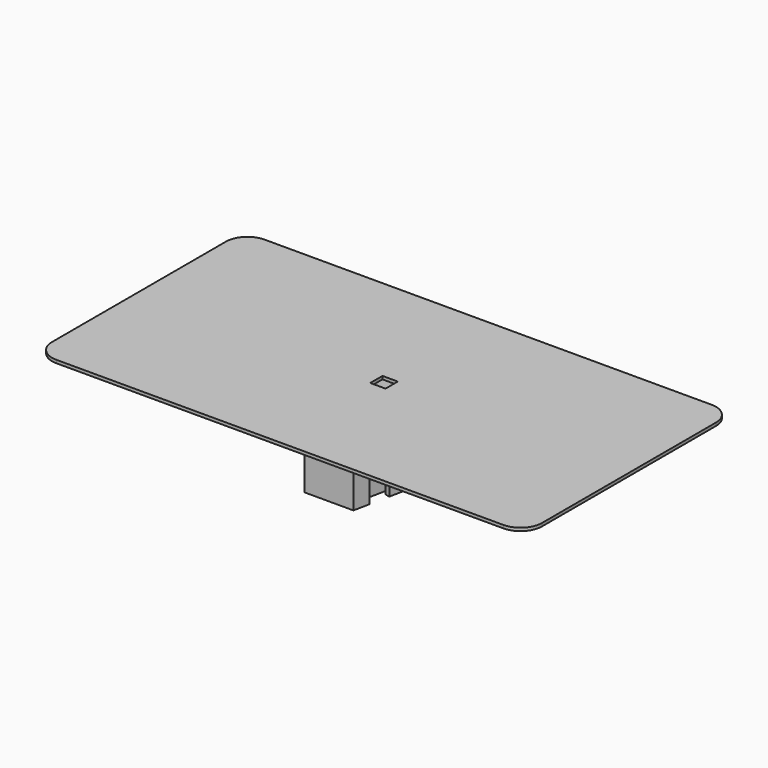
from build123d import *

# Parameters (mm, degrees)
F0_R      = 8
F1_DEPTH  = 1
F3_R      = 8
F4_DEPTH  = 24.1
F7_DEPTH  = 8.7145
F9_DEPTH  = 8.175
F11_DEPTH = 8.715
F13_DEPTH = 8.715
F14_W     = 5
F14_H     = 5
F15_DEPTH = 25
F17_DEPTH = 34.8
F18_R     = 1
F20_R     = 1.5
F21_DEPTH = 8.88


# Not quite as in the source:
# - a feature of the source that left no trace in its solid (it failed there, or was rolled back) is left out


with BuildPart() as f1:
    # F0 (on Top) → F1 (new body)
    with BuildSketch(Plane.XY):
        with BuildLine():
            Line((-73, -42.5), (73, -42.5))
            ThreePointArc((73, -42.5), (77.9497474683, -40.4497474683), (80, -35.5))
            Line((80, -35.5), (80, 35.5))
            ThreePointArc((80, 35.5), (77.9497474683, 40.4497474683), (73, 42.5))
            Line((73, 42.5), (-73, 42.5))
            ThreePointArc((-73, 42.5), (-77.9497474683, 40.4497474683), (-80, 35.5))
            Line((-80, 35.5), (-80, -35.5))
            ThreePointArc((-80, -35.5), (-77.9497474683, -40.4497474683), (-73, -42.5))
        make_face()
        Circle(F0_R, mode=Mode.SUBTRACT)
        Circle(F0_R)
    extrude(amount=F1_DEPTH)

    # F3 (on face) → F4 (join)
    with BuildSketch(Plane(origin=(0, 0, 0), x_dir=(1, 0, 0), z_dir=(0, 0, -1))):
        Polygon((10.7943351377, -8.8776162038), (12, -3), (12, 3), (11.1962234251, 6.9184108026), (10.3924468502, 10.8368216051), (8.9230427993, 10.5354053895), (9.3249310867, 8.5761999883), (7.8555270357, 8.2747837727), (5.7456135267, 18.5606121294), (7.2150175776, 18.862028345), (7.6169058651, 16.9028229437), (9.086309916, 17.2042391593), (8, 22.5), (-8, 22.5), (-9.086309916, 17.2042391593), (-7.6169058651, 16.9028229437), (-7.2150175776, 18.862028345), (-5.7456135267, 18.5606121294), (-7.8555270357, 8.2747837727), (-9.3249310867, 8.5761999883), (-8.9230427993, 10.5354053895), (-10.3924468502, 10.8368216051), (-11.1962234251, 6.9184108026), (-12, 3), (-12, -3), (-11.1962234251, -6.9184108026), (-10.3924468502, -10.8368216051), (-8.9230427993, -10.5354053895), (-9.3249310867, -8.5761999883), (-7.8555270357, -8.2747837727), (-5.7456135267, -18.5606121294), (-7.2150175776, -18.862028345), (-7.6169058651, -16.9028229437), (-9.086309916, -17.2042391593), (-8, -22.5), (8, -22.5), (8.9858378442, -17.6940405096), (9.086309916, -17.2042391593), (7.6169058651, -16.9028229437), (7.2150175776, -18.862028345), (5.7456135267, -18.5606121294), (7.8555270357, -8.2747837727), (9.3249310867, -8.5761999883), (8.9230427993, -10.5354053895), (10.3924468502, -10.8368216051), align=None)
        Circle(F3_R, mode=Mode.SUBTRACT)
    extrude(amount=F4_DEPTH)

    # F6 (on face) → F7 (cut)
    with BuildSketch(Plane(origin=(9.1671855889, 1.8804483259, 0), x_dir=(-0.2009441437, 0.9796027006, 0), z_dir=(0.9796027006, 0.2009441437, 0))):
        with BuildLine():
            ThreePointArc((13.2774783773, -11.45), (12.838138549, -10.3893398282), (11.7774783773, -9.95))
            ThreePointArc((11.7774783773, -9.95), (10.7168182055, -12.5106601718), (13.2774783773, -11.45))
        make_face()
    extrude(amount=-F7_DEPTH, mode=Mode.SUBTRACT)

    # F8 (on face) → F9 (cut)
    with BuildSketch(Plane(origin=(-9.1671855889, 1.8804483259, 0), x_dir=(-0.2009441437, -0.9796027006, 0), z_dir=(-0.9796027006, 0.2009441437, 0))):
        with BuildLine():
            ThreePointArc((-10.2774783773, -11.45), (-10.7168182055, -10.3893398282), (-11.7774783773, -9.95))
            ThreePointArc((-11.7774783773, -9.95), (-12.838138549, -12.5106601718), (-10.2774783773, -11.45))
        make_face()
    extrude(amount=-F9_DEPTH, mode=Mode.SUBTRACT)

    # F10 (on face) → F11 (cut)
    with BuildSketch(Plane(origin=(-9.1671855889, -1.8804483259, 0), x_dir=(0.2009441437, -0.9796027006, 0), z_dir=(-0.9796027006, -0.2009441437, 0))):
        with BuildLine():
            ThreePointArc((11.7774783773, -9.95), (10.7168182055, -12.5106601718), (13.2774783773, -11.45))
            ThreePointArc((13.2774783773, -11.45), (12.838138549, -10.3893398282), (11.7774783773, -9.95))
        make_face()
    extrude(amount=-F11_DEPTH, mode=Mode.SUBTRACT)

    # F12 (on face) → F13 (cut)
    with BuildSketch(Plane(origin=(9.1671855889, -1.8804483259, 0), x_dir=(0.2009441437, 0.9796027006, 0), z_dir=(0.9796027006, -0.2009441437, 0))):
        with BuildLine():
            ThreePointArc((-11.7774783773, -9.95), (-12.838138549, -12.5106601718), (-10.2774783773, -11.45))
            ThreePointArc((-10.2774783773, -11.45), (-10.7168182055, -10.3893398282), (-11.7774783773, -9.95))
        make_face()
    extrude(amount=-F13_DEPTH, mode=Mode.SUBTRACT)

    # F14 (on face) → F15 (cut)
    with BuildSketch(Plane(origin=(0, 0, 0), x_dir=(1, 0, 0), z_dir=(0, 0, -1))):
        Rectangle(F14_W, F14_H)
    extrude(amount=-F15_DEPTH, mode=Mode.SUBTRACT)

    # F16 (on face) → F17 (cut)
    with BuildSketch(Plane.XZ.offset(22.5)):
        with BuildLine():
            ThreePointArc((0, -10.55), (-1.5, -12.05), (0, -13.55))
            Line((0, -13.55), (0, -12.05))
            Line((0, -12.05), (0, -10.55))
        make_face()
        with BuildLine():
            Line((0, -12.05), (0, -13.55))
            ThreePointArc((0, -13.55), (1.0606601718, -13.1106601718), (1.5, -12.05))
            ThreePointArc((1.5, -12.05), (1.0606601718, -10.9893398282), (0, -10.55))
            Line((0, -10.55), (0, -12.05))
        make_face()
    extrude(amount=-F17_DEPTH, mode=Mode.SUBTRACT)

    # F18
    f18_edges = [f1.edges().sort_by_distance(p)[0] for p in [
        (8, 0, -12.05),
        (0, -8, -10.55),
        (0, 8, -10.55),
    ]]
    fillet(f18_edges, radius=F18_R)

    # F20 (on face) → F21 (join)
    with BuildSketch(Plane.XZ.offset(22.5)):
        with Locations((0, -12.05)):
            Circle(F20_R)
    extrude(amount=-F21_DEPTH)


solid = f1.part
